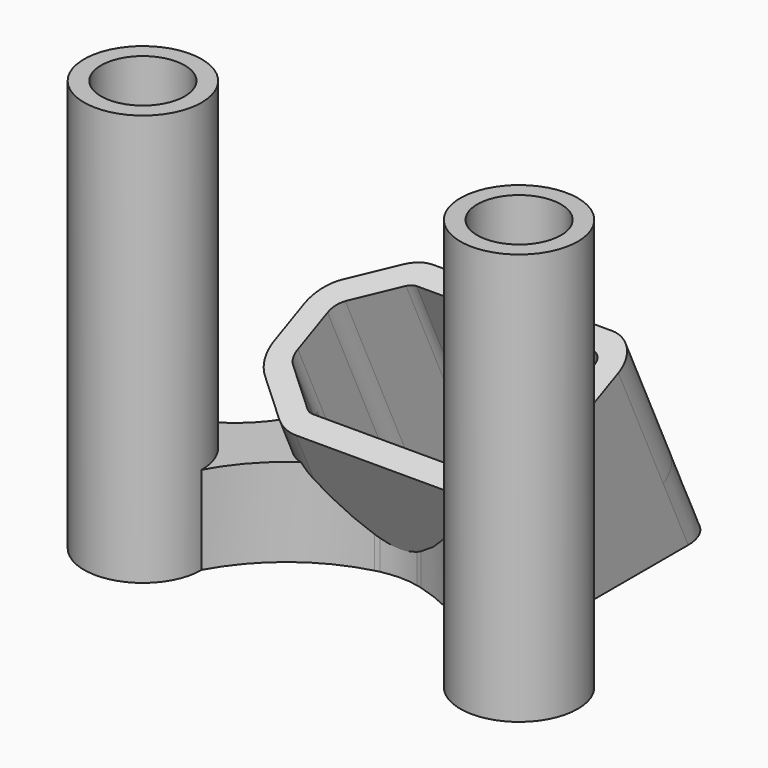
from build123d import *

# Parameters (mm, degrees)
F0_R      = 4
F0_R_2    = 2.85
F2_DEPTH  = 28
F4_DEPTH  = 6
F7_DEPTH  = 50
F8_REACH  = 28.3339417877
F9_DEPTH  = 9
F10_DEPTH = 6
F12_DEPTH = 50


# Not quite as in the source:
# - a feature names something its author has since deleted; it is built from what else it names


with BuildPart() as f2:
    # F0 (on Top) → F2 (new body)
    with BuildSketch(Plane.XY):
        with Locations((-12.8, 0)):
            Circle(F0_R)
        with Locations((-12.8, 0)):
            Circle(F0_R_2, mode=Mode.SUBTRACT)
    extrude(amount=F2_DEPTH)


with BuildPart() as f2b:
    # F0 (on Top) → F2, piece 2 (new body)
    with BuildSketch(Plane.XY):
        with Locations((12.8, 0)):
            Circle(F0_R)
        with Locations((12.8, 0)):
            Circle(F0_R_2, mode=Mode.SUBTRACT)
    extrude(amount=F2_DEPTH)


with BuildPart() as f4:
    # F3 (on Top) → F4 (new body)
    with BuildSketch(Plane.XY):
        with BuildLine():
            Line((7.5, 18.35), (-4.6556847597, 18.35))
            ThreePointArc((-4.6556847597, 18.35), (-5.5021347681, 18.2083576597), (-6.2563592688, 17.7988633717))
            Line((-6.2563592688, 17.7988633717), (-8.8006745091, 15.8111170902))
            ThreePointArc((-8.8006745091, 15.8111170902), (-9.5368519127, 14.9020445494), (-9.8, 13.7622537185))
            Line((-9.8, 13.7622537185), (-9.8, 12.5))
            Line((-9.8, 12.5), (-9.8, 11.2377462815))
            ThreePointArc((-9.8, 11.2377462815), (-9.5368519127, 10.0979554506), (-8.8006745091, 9.1888829098))
            Line((-8.8006745091, 9.1888829098), (-6.2563592688, 7.2011366283))
            ThreePointArc((-6.2563592688, 7.2011366283), (-5.5021347681, 6.7916423403), (-4.6556847597, 6.65))
            Line((-4.6556847597, 6.65), (7.5, 6.65))
            ThreePointArc((7.5, 6.65), (8.9849242405, 7.2650757595), (9.6, 8.75))
            Line((9.6, 8.75), (9.6, 12.5))
            Line((9.6, 12.5), (9.6, 16.25))
            ThreePointArc((9.6, 16.25), (8.9849242405, 17.7349242405), (7.5, 18.35))
        make_face()
    extrude(amount=F4_DEPTH)

    # F6 (on offset) → F7 (cut)
    with BuildSketch(Plane.YZ.offset(9.6)):
        Polygon((6.4474307001, 6.8065319635), (6.4474307001, 0), (21.0440856005, 6.8065319635), align=None)
    extrude(amount=-F7_DEPTH, mode=Mode.SUBTRACT)

    f8_end = Plane(origin=(0.3975429919, 12.5, 0), x_dir=(-1, 0, 0), z_dir=(0, 0, -1))
    # F7_face (on face) → F8 (join, up to a plane its end follows)
    with BuildSketch(Plane(origin=(0.3975429919, 12.5, 2.8223594161), x_dir=(1, 0, 0), z_dir=(0, -0.4226182617, 0.906307787))):
        with BuildLine():
            Line((9.2024570081, -4.1376671961), (9.2024570081, 4.1376671961))
            add(Edge.make_bspline(
                [(7.1024570081, 6.4547608259), (9.2024570081, 6.4547608259), (9.2024570081, 4.1376671961)],
                knots=[3.1415926536, 3.1415926536, 3.1415926536, 4.7123889804, 4.7123889804, 4.7123889804], degree=2, weights=[1, 0.7071067812, 1]))
            Line((7.1024570081, 6.4547608259), (-5.0532277516, 6.4547608259))
            add(Edge.make_bspline(
                [(-6.6539022607, 5.8466488399), (-5.9484473765, 6.4547608259), (-5.0532277516, 6.4547608259)],
                knots=[2.4783896609, 2.4783896609, 2.4783896609, 3.1415926536, 3.1415926536, 3.1415926536], degree=2, weights=[1, 0.9455221768, 1]))
            Line((-6.6539022607, 5.8466488399), (-9.198217501, 3.6534134844))
            add(Edge.make_bspline(
                [(-10.1975429919, 1.3927428811), (-10.1975429919, 2.7919809215), (-9.198217501, 3.6534134844)],
                knots=[1.5707963268, 1.5707963268, 1.5707963268, 2.4783896609, 2.4783896609, 2.4783896609], degree=2, weights=[1, 0.8987891972, 1]))
            Line((-10.1975429919, 1.3927428811), (-10.1975429919, -1.3927428811))
            add(Edge.make_bspline(
                [(-9.198217501, -3.6534134844), (-10.1975429919, -2.7919809215), (-10.1975429919, -1.3927428811)],
                knots=[0.6632029927, 0.6632029927, 0.6632029927, 1.5707963268, 1.5707963268, 1.5707963268], degree=2, weights=[1, 0.8987891972, 1]))
            Line((-9.198217501, -3.6534134844), (-6.6539022607, -5.8466488399))
            add(Edge.make_bspline(
                [(-5.0532277516, -6.4547608259), (-5.9484473765, -6.4547608259), (-6.6539022607, -5.8466488399)],
                knots=[0, 0, 0, 0.6632029927, 0.6632029927, 0.6632029927], degree=2, weights=[1, 0.9455221768, 1]))
            Line((-5.0532277516, -6.4547608259), (7.1024570081, -6.4547608259))
            add(Edge.make_bspline(
                [(9.2024570081, -4.1376671961), (9.2024570081, -6.4547608259), (7.1024570081, -6.4547608259)],
                knots=[4.7123889804, 4.7123889804, 4.7123889804, 6.2831853072, 6.2831853072, 6.2831853072], degree=2, weights=[1, 0.7071067812, 1]))
        make_face()
    f8_long = extrude(amount=-F8_REACH, mode=Mode.PRIVATE)
    add(split(f8_long, bisect_by=f8_end, keep=Keep.BOTTOM, mode=Mode.PRIVATE))

    # F9 (add): a face of the model
    f9_faces = [f4.faces().sort_by_distance(p)[0] for p in [
        (0.3975429919, 12.5, 2.8223594161),
    ]]
    extrude(f9_faces, amount=F9_DEPTH)


with BuildPart() as f10:
    # F1 (on Top) → F10 (new body)
    with BuildSketch(Plane.XY):
        with BuildLine():
            ThreePointArc((-1.2596207883, 5.7537340458), (0, 5.89), (1.2596207883, 5.7537340458))
            ThreePointArc((1.2596207883, 5.7537340458), (1.4230201919, 5.7155151591), (1.5852645107, 5.6726569111))
            ThreePointArc((1.5852645107, 5.6726569111), (5.7790969207, 3.5822201075), (8.8, 0))
            ThreePointArc((8.8, 0), (10.1071311565, 2.9577791317), (13.174228696, 3.9824556348))
            ThreePointArc((13.174228696, 3.9824556348), (9.8667045598, 6.1744840875), (8, 9.6759293228))
            Line((8, 9.6759293228), (8, 8.75))
            ThreePointArc((8, 8.75), (7.8535533906, 8.3964466094), (7.5, 8.25))
            Line((7.5, 8.25), (-4.6556847597, 8.25))
            ThreePointArc((-4.6556847597, 8.25), (-4.9812424552, 8.3044778232), (-5.2713288016, 8.4619756263))
            Line((-5.2713288016, 8.4619756263), (-7.815644042, 10.4497219078))
            ThreePointArc((-7.815644042, 10.4497219078), (-7.9140380275, 10.5376393644), (-8, 10.6377462815))
            Line((-8, 10.6377462815), (-8, 9.6759293228))
            ThreePointArc((-8, 9.6759293228), (-9.8667045598, 6.1744840875), (-13.174228696, 3.9824556348))
            ThreePointArc((-13.174228696, 3.9824556348), (-10.1071311565, 2.9577791317), (-8.8, 0))
            ThreePointArc((-8.8, 0), (-5.7790969207, 3.5822201075), (-1.5852645107, 5.6726569111))
            ThreePointArc((-1.5852645107, 5.6726569111), (-1.4230201919, 5.7155151591), (-1.2596207883, 5.7537340458))
        make_face()
    extrude(amount=F10_DEPTH)


with BuildPart() as f12_tool:
    # F11 (on face) → F12 (new body)
    with BuildSketch(Plane(origin=(0, -2.6520132898, 5.6872608532), x_dir=(1, 0, 0), z_dir=(0, -0.4226182617, 0.906307787))):
        with BuildLine():
            ThreePointArc((8, 16.6592951645), (7.8626590068, 17.0963944879), (7.5, 17.3763887943))
            Line((7.5, 17.3763887943), (-4.6556847597, 17.3763887943))
            ThreePointArc((-4.6556847597, 17.3763887943), (-4.9522690953, 17.3133448608), (-5.2116940879, 17.1563879273))
            Line((-5.2116940879, 17.1563879273), (-7.7560093283, 14.9631525718))
            ThreePointArc((-7.7560093283, 14.9631525718), (-8.0844304273, 14.4838159341), (-8.2, 13.9143708495))
            Line((-8.2, 13.9143708495), (-8.2, 11.1288850873))
            ThreePointArc((-8.2, 11.1288850873), (-8.1004846181, 10.5526436305), (-7.7560093283, 10.080103365))
            Line((-7.7560093283, 10.080103365), (-5.2116940879, 7.8868680095))
            ThreePointArc((-5.2116940879, 7.8868680095), (-4.9546608267, 7.7238664411), (-4.6556847597, 7.6668671425))
            Line((-4.6556847597, 7.6668671425), (7.5, 7.6668671425))
            ThreePointArc((7.5, 7.6668671425), (7.8626590068, 7.9468614489), (8, 8.3839607723))
            Line((8, 8.3839607723), (8, 16.6592951645))
        make_face()
    extrude(amount=-F12_DEPTH)


with BuildPart() as f4_1:
    add(f4.part)

    # F12: cut by f12_tool
    add(f12_tool.part, mode=Mode.SUBTRACT)


with BuildPart() as f10_1:
    add(f10.part)

    # F12: cut by f12_tool
    add(f12_tool.part, mode=Mode.SUBTRACT)


solid = Compound([f2.part, f2b.part, f4_1.part, f10_1.part])
